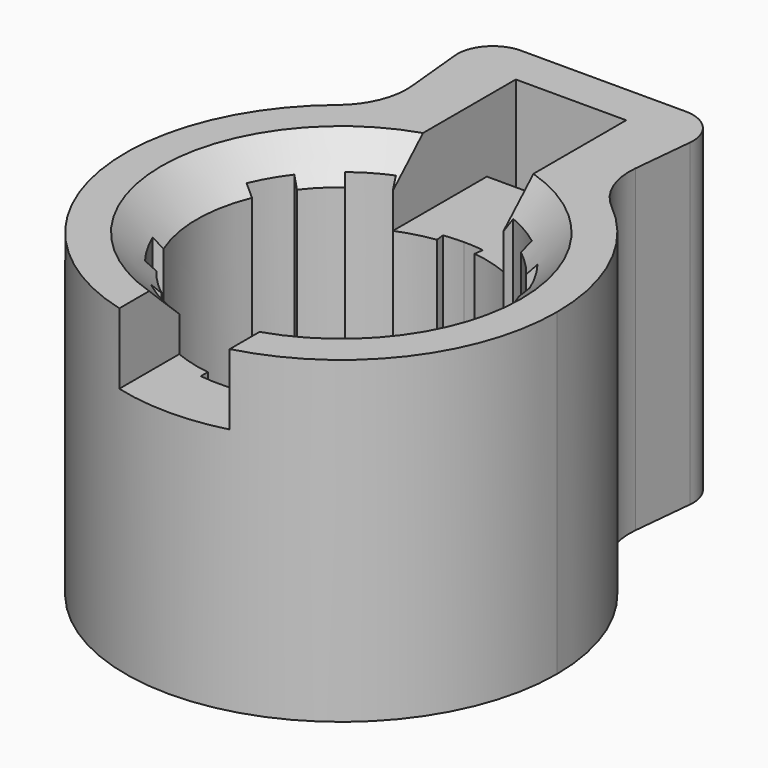
from build123d import *

# Parameters (mm, degrees)
F0_W         = 3.9597223513
F0_H         = 1.2967120856
F1_DEPTH     = 11.43
F2_R         = 2.54
F4_DEPTH     = 11.43
F5_DEPTH     = 2.54
F6_T2_ANGLE  = 117.2359685867
F6_T4_ANGLE  = 87.2295221482
F6_T6_ANGLE  = 87.2295221482
F6_T8_ANGLE  = 87.2295221482
F6_T10_ANGLE = 87.2295221482
F6_T12_ANGLE = 87.2295221482
F6_T14_ANGLE = 87.2295221482
F6_T16_ANGLE = 72.2652313511
F6_T18_ANGLE = 72.2652313511
F6_T20_ANGLE = 72.2652313511
F6_T22_ANGLE = 72.2652313511
F7_R         = 1.27


# Not quite as in the source:
# - a fillet or chamfer that OpenCascade refuses, or shapes differently, is made with other operations: its cross-section is extruded or revolved along the edge and cut away or added
# - a feature names something its author has since deleted; it is built from what else it names


with BuildPart() as f1:
    # F0 (on Top) → F1 (new body)
    with BuildSketch(Plane.XY):
        with BuildLine():
            ThreePointArc((-3.8608, 6.7017624436), (-3.8703236977, -6.6962669425), (7.7343, 0))
            ThreePointArc((7.7343, 0), (6.6962669425, 3.8703236977), (3.8608, 6.7017624436))
            ThreePointArc((3.8608, 6.7017624436), (1.9982436316, 7.4717078957), (0, 7.7343))
            ThreePointArc((0, 7.7343), (-1.9982436316, 7.4717078957), (-3.8608, 6.7017624436))
        make_face()
        with BuildLine():
            ThreePointArc((-0.7177765836, 5.4520544372), (-0.3596583479, 5.4873260048), (0, 5.4991))
            ThreePointArc((0, 5.4991), (0.3596583479, 5.4873260048), (0.7177765836, 5.4520544372))
            ThreePointArc((0.7177765836, 5.4520544372), (1.4232718109, 5.3117227113), (2.1044144629, 5.0805059372))
            ThreePointArc((2.1044144629, 5.0805059372), (2.74955, 4.762360298), (3.3476399743, 4.3627293536))
            ThreePointArc((3.3476399743, 4.3627293536), (3.8884509004, 3.8884509004), (4.3627293536, 3.3476399743))
            ThreePointArc((4.3627293536, 3.3476399743), (4.762360298, 2.74955), (5.0805059372, 2.1044144629))
            ThreePointArc((5.0805059372, 2.1044144629), (5.3117227113, 1.4232718109), (5.4520544372, 0.7177765836))
            ThreePointArc((5.4520544372, 0.7177765836), (5.4873260048, 0.3596583479), (5.4991, 0))
            ThreePointArc((5.4991, 0), (5.4873260048, -0.3596583479), (5.4520544372, -0.7177765836))
            ThreePointArc((5.4520544372, -0.7177765836), (5.3117227113, -1.4232718109), (5.0805059372, -2.1044144629))
            ThreePointArc((5.0805059372, -2.1044144629), (4.762360298, -2.74955), (4.3627293536, -3.3476399743))
            ThreePointArc((4.3627293536, -3.3476399743), (3.8884509004, -3.8884509004), (3.3476399743, -4.3627293536))
            ThreePointArc((3.3476399743, -4.3627293536), (2.74955, -4.762360298), (2.1044144629, -5.0805059372))
            ThreePointArc((2.1044144629, -5.0805059372), (1.4232718109, -5.3117227113), (0.7177765836, -5.4520544372))
            ThreePointArc((0.7177765836, -5.4520544372), (0.0208895376, -5.4990603231), (-0.6763345176, -5.4573503122))
            ThreePointArc((-0.6763345176, -5.4573503122), (-1.4030837979, -5.3170909966), (-2.1044144629, -5.0805059372))
            ThreePointArc((-2.1044144629, -5.0805059372), (-2.74955, -4.762360298), (-3.3476399743, -4.3627293536))
            ThreePointArc((-3.3476399743, -4.3627293536), (-3.8884509004, -3.8884509004), (-4.3627293536, -3.3476399743))
            ThreePointArc((-4.3627293536, -3.3476399743), (-4.762360298, -2.74955), (-5.0805059372, -2.1044144629))
            ThreePointArc((-5.0805059372, -2.1044144629), (-5.4991, 0), (-5.0805059372, 2.1044144629))
            ThreePointArc((-5.0805059372, 2.1044144629), (-4.762360298, 2.74955), (-4.3627293536, 3.3476399743))
            ThreePointArc((-4.3627293536, 3.3476399743), (-3.8884509004, 3.8884509004), (-3.3476399743, 4.3627293536))
            ThreePointArc((-3.3476399743, 4.3627293536), (-2.74955, 4.762360298), (-2.1044144629, 5.0805059372))
            ThreePointArc((-2.1044144629, 5.0805059372), (-1.4232718109, 5.3117227113), (-0.7177765836, 5.4520544372))
        make_face(mode=Mode.SUBTRACT)
        with BuildLine():
            ThreePointArc((0, 7.7343), (1.9982436316, 7.4717078957), (3.8608, 6.7017624436))
            Line((3.8608, 6.7017624436), (4.3561, 11.75755891))
            Line((4.3561, 11.75755891), (-4.3561, 11.75755891))
            Line((-4.3561, 11.75755891), (-3.8608, 6.7017624436))
            ThreePointArc((-3.8608, 6.7017624436), (-1.9982436316, 7.4717078957), (0, 7.7343))
        make_face()
        with Locations((0, 9.6516758204)):
            Rectangle(F0_W, F0_H, mode=Mode.SUBTRACT)
    extrude(amount=F1_DEPTH)

    # F2
    f2_edges = [f1.edges().sort_by_distance(p)[0] for p in [
        (3.8608, 6.701762, 5.715),
        (-3.8608, 6.701762, 5.715),
    ]]
    fillet(f2_edges, radius=F2_R)

    # F0 (on Top) → F4 (join)
    with BuildSketch(Plane.XY):
        with BuildLine():
            Line((-4.3627293536, 3.3476399743), (-4.1108396681, 3.1543582206))
            ThreePointArc((-4.1108396681, 3.1543582206), (-3.6639444974, 3.6639444974), (-3.1543582206, 4.1108396681))
            Line((-3.1543582206, 4.1108396681), (-3.3476399743, 4.3627293536))
            ThreePointArc((-3.3476399743, 4.3627293536), (-3.8884509004, 3.8884509004), (-4.3627293536, 3.3476399743))
        make_face()
        with BuildLine():
            Line((-0.6763345176, 5.1372706937), (-0.7177765836, 5.4520544372))
            ThreePointArc((-0.7177765836, 5.4520544372), (-1.4232718109, 5.3117227113), (-2.1044144629, 5.0805059372))
            Line((-2.1044144629, 5.0805059372), (-1.9829124731, 4.7871741857))
            ThreePointArc((-1.9829124731, 4.7871741857), (-1.3410967641, 5.0050412615), (-0.6763345176, 5.1372706937))
        make_face()
        with BuildLine():
            ThreePointArc((2.1044144629, 5.0805059372), (1.4232718109, 5.3117227113), (0.7177765836, 5.4520544372))
            Line((0.7177765836, 5.4520544372), (0.6763345176, 5.1372706937))
            ThreePointArc((0.6763345176, 5.1372706937), (1.3410967641, 5.0050412615), (1.9829124731, 4.7871741857))
            Line((1.9829124731, 4.7871741857), (2.1044144629, 5.0805059372))
        make_face()
        with BuildLine():
            Line((3.3476399743, 4.3627293536), (3.1543582206, 4.1108396681))
            ThreePointArc((3.1543582206, 4.1108396681), (3.6639444974, 3.6639444974), (4.1108396681, 3.1543582206))
            Line((4.1108396681, 3.1543582206), (4.3627293536, 3.3476399743))
            ThreePointArc((4.3627293536, 3.3476399743), (3.8884509004, 3.8884509004), (3.3476399743, 4.3627293536))
        make_face()
        with BuildLine():
            ThreePointArc((4.7871741857, 1.9829124731), (5.0050412615, 1.3410967641), (5.1372706937, 0.6763345176))
            Line((5.1372706937, 0.6763345176), (5.4520544372, 0.7177765836))
            ThreePointArc((5.4520544372, 0.7177765836), (5.3117227113, 1.4232718109), (5.0805059372, 2.1044144629))
            Line((5.0805059372, 2.1044144629), (4.7871741857, 1.9829124731))
        make_face()
        with BuildLine():
            ThreePointArc((-4.7871741857, -1.9829124731), (-5.1816, 0), (-4.7871741857, 1.9829124731))
            Line((-4.7871741857, 1.9829124731), (-5.0805059372, 2.1044144629))
            ThreePointArc((-5.0805059372, 2.1044144629), (-5.4991, 0), (-5.0805059372, -2.1044144629))
            Line((-5.0805059372, -2.1044144629), (-4.7871741857, -1.9829124731))
        make_face()
        with BuildLine():
            ThreePointArc((-3.1543582206, -4.1108396681), (-3.6639444974, -3.6639444974), (-4.1108396681, -3.1543582206))
            Line((-4.1108396681, -3.1543582206), (-4.3627293536, -3.3476399743))
            ThreePointArc((-4.3627293536, -3.3476399743), (-3.8884509004, -3.8884509004), (-3.3476399743, -4.3627293536))
            Line((-3.3476399743, -4.3627293536), (-3.1543582206, -4.1108396681))
        make_face()
        with BuildLine():
            ThreePointArc((-0.6763345176, -5.1372706937), (-1.3410967641, -5.0050412615), (-1.9829124731, -4.7871741857))
            Line((-1.9829124731, -4.7871741857), (-2.1044144629, -5.0805059372))
            ThreePointArc((-2.1044144629, -5.0805059372), (-1.4030837979, -5.3170909966), (-0.6763345176, -5.4573503122))
            Line((-0.6763345176, -5.4573503122), (-0.6763345176, -5.1372706937))
        make_face()
        with BuildLine():
            ThreePointArc((1.9829124731, -4.7871741857), (1.3410967641, -5.0050412615), (0.6763345176, -5.1372706937))
            Line((0.6763345176, -5.1372706937), (0.7177765836, -5.4520544372))
            ThreePointArc((0.7177765836, -5.4520544372), (1.4232718109, -5.3117227113), (2.1044144629, -5.0805059372))
            Line((2.1044144629, -5.0805059372), (1.9829124731, -4.7871741857))
        make_face()
        with BuildLine():
            ThreePointArc((4.1108396681, -3.1543582206), (3.6639444974, -3.6639444974), (3.1543582206, -4.1108396681))
            Line((3.1543582206, -4.1108396681), (3.3476399743, -4.3627293536))
            ThreePointArc((3.3476399743, -4.3627293536), (3.8884509004, -3.8884509004), (4.3627293536, -3.3476399743))
            Line((4.3627293536, -3.3476399743), (4.1108396681, -3.1543582206))
        make_face()
        with BuildLine():
            ThreePointArc((5.1372706937, -0.6763345176), (5.0050412615, -1.3410967641), (4.7871741857, -1.9829124731))
            Line((4.7871741857, -1.9829124731), (5.0805059372, -2.1044144629))
            ThreePointArc((5.0805059372, -2.1044144629), (5.3117227113, -1.4232718109), (5.4520544372, -0.7177765836))
            Line((5.4520544372, -0.7177765836), (5.1372706937, -0.6763345176))
        make_face()
    extrude(amount=F4_DEPTH)

    # F3 (on face) → F5 (cut)
    with BuildSketch(Plane.XY.offset(11.43)):
        with BuildLine():
            Line((1.9798611756, 5.1303265525), (1.9798611756, 9.0033197775))
            Line((1.9798611756, 9.0033197775), (-1.9798611756, 9.0033197775))
            Line((-1.9798611756, 9.0033197775), (-1.9798611756, 5.1303265525))
            ThreePointArc((-1.9798611756, 5.1303265525), (0, 5.4991), (1.9798611756, 5.1303265525))
        make_face()
        with BuildLine():
            Line((1.9798611756, -5.1303265525), (1.9798611756, 5.1303265525))
            ThreePointArc((1.9798611756, 5.1303265525), (0, 5.4991), (-1.9798611756, 5.1303265525))
            Line((-1.9798611756, 5.1303265525), (-1.9798611756, -5.1303265525))
            ThreePointArc((-1.9798611756, -5.1303265525), (0, -5.4991), (1.9798611756, -5.1303265525))
        make_face()
        with BuildLine():
            Line((1.9798611756, -7.4765999101), (1.9798611756, -5.1303265525))
            ThreePointArc((1.9798611756, -5.1303265525), (0, -5.4991), (-1.9798611756, -5.1303265525))
            Line((-1.9798611756, -5.1303265525), (-1.9798611756, -7.4765999101))
            ThreePointArc((-1.9798611756, -7.4765999101), (0, -7.7343), (1.9798611756, -7.4765999101))
        make_face()
    extrude(amount=-F5_DEPTH, mode=Mode.SUBTRACT)

    # F6: chamfer of 1.27 on 11 edges, made by hand

    # F6_s1 → F6_t2 (revolve, cut)
    with BuildSketch(Plane(origin=(0, 0, 0), x_dir=(0, 0, 1), z_dir=(0.8537142924, -0.5207416893, 0))):
        Polygon((11.43, 6.4516), (10.16, 5.1816), (11.43, 5.1816), align=None)
    revolve(axis=Axis((0, 0, 11.43), (0, 0, -1)), revolution_arc=F6_T2_ANGLE, mode=Mode.SUBTRACT)

    # F6_s3 → F6_t4 (revolve, cut)
    with BuildSketch(Plane(origin=(0, 0, 0), x_dir=(0, 0, 1), z_dir=(0.9997077511, -0.0241746249, 0))):
        Polygon((11.43, 6.4516), (10.16, 5.1816), (11.43, 5.1816), align=None)
    revolve(axis=Axis((0, 0, 11.43), (0, 0, -1)), revolution_arc=F6_T4_ANGLE, mode=Mode.SUBTRACT)

    # F6_s5 → F6_t6 (revolve, cut)
    with BuildSketch(Plane(origin=(0, 0, 0), x_dir=(0, 0, 1), z_dir=(-0.0241746249, -0.9997077511, 0))):
        Polygon((11.43, 6.4516), (10.16, 5.1816), (11.43, 5.1816), align=None)
    revolve(axis=Axis((0, 0, 11.43), (0, 0, -1)), revolution_arc=F6_T6_ANGLE, mode=Mode.SUBTRACT)

    # F6_s7 → F6_t8 (revolve, cut)
    with BuildSketch(Plane(origin=(0, 0, 0), x_dir=(0, 0, 1), z_dir=(-0.9997077511, 0.0241746249, 0))):
        Polygon((11.43, 6.4516), (10.16, 5.1816), (11.43, 5.1816), align=None)
    revolve(axis=Axis((0, 0, 11.43), (0, 0, -1)), revolution_arc=F6_T8_ANGLE, mode=Mode.SUBTRACT)

    # F6_s9 → F6_t10 (revolve, cut)
    with BuildSketch(Plane(origin=(0, 0, 0), x_dir=(0, 0, 1), z_dir=(-0.8536849963, 0.5207897148, 0))):
        Polygon((11.43, 6.4516), (10.16, 5.1816), (11.43, 5.1816), align=None)
    revolve(axis=Axis((0, 0, 11.43), (0, 0, -1)), revolution_arc=F6_T10_ANGLE, mode=Mode.SUBTRACT)

    # F6_s11 → F6_t12 (revolve, cut)
    with BuildSketch(Plane(origin=(0, 0, 0), x_dir=(0, 0, 1), z_dir=(-0.4789180362, 0.8778596212, 0))):
        Polygon((11.43, 6.4516), (10.16, 5.1816), (11.43, 5.1816), align=None)
    revolve(axis=Axis((0, 0, 11.43), (0, 0, -1)), revolution_arc=F6_T12_ANGLE, mode=Mode.SUBTRACT)

    # F6_s13 → F6_t14 (revolve, cut)
    with BuildSketch(Plane(origin=(0, 0, 0), x_dir=(0, 0, 1), z_dir=(0.0241746249, 0.9997077511, 0))):
        Polygon((11.43, 6.4516), (10.16, 5.1816), (11.43, 5.1816), align=None)
    revolve(axis=Axis((0, 0, 11.43), (0, 0, -1)), revolution_arc=F6_T14_ANGLE, mode=Mode.SUBTRACT)

    # F6_s15 → F6_t16 (revolve, cut)
    with BuildSketch(Plane(origin=(0, 0, 0), x_dir=(0, 0, 1), z_dir=(0.9717518339, 0.2360050283, 0))):
        Polygon((11.43, 6.4516), (10.16, 5.1816), (11.43, 5.1816), align=None)
    revolve(axis=Axis((0, 0, 11.43), (0, 0, -1)), revolution_arc=F6_T16_ANGLE, mode=Mode.SUBTRACT)

    # F6_s17 → F6_t18 (revolve, cut)
    with BuildSketch(Plane(origin=(0, 0, 0), x_dir=(0, 0, 1), z_dir=(-0.5207957174, -0.8536813344, 0))):
        Polygon((11.43, 6.4516), (10.16, 5.1816), (11.43, 5.1816), align=None)
    revolve(axis=Axis((0, 0, 11.43), (0, 0, -1)), revolution_arc=F6_T18_ANGLE, mode=Mode.SUBTRACT)

    # F6_s19 → F6_t20 (revolve, cut)
    with BuildSketch(Plane(origin=(0, 0, 0), x_dir=(0, 0, 1), z_dir=(-0.9717518339, -0.2360050283, 0))):
        Polygon((11.43, 6.4516), (10.16, 5.1816), (11.43, 5.1816), align=None)
    revolve(axis=Axis((0, 0, 11.43), (0, 0, -1)), revolution_arc=F6_T20_ANGLE, mode=Mode.SUBTRACT)

    # F6_s21 → F6_t22 (revolve, cut)
    with BuildSketch(Plane(origin=(0, 0, 0), x_dir=(0, 0, 1), z_dir=(0.5207957174, 0.8536813344, 0))):
        Polygon((11.43, 6.4516), (10.16, 5.1816), (11.43, 5.1816), align=None)
    revolve(axis=Axis((0, 0, 11.43), (0, 0, -1)), revolution_arc=F6_T22_ANGLE, mode=Mode.SUBTRACT)

    # F7
    f7_edges = [f1.edges().sort_by_distance(p)[0] for p in [
        (-4.3561, 11.757559, 5.715),
        (4.3561, 11.757559, 5.715),
    ]]
    fillet(f7_edges, radius=F7_R)


solid = f1.part
